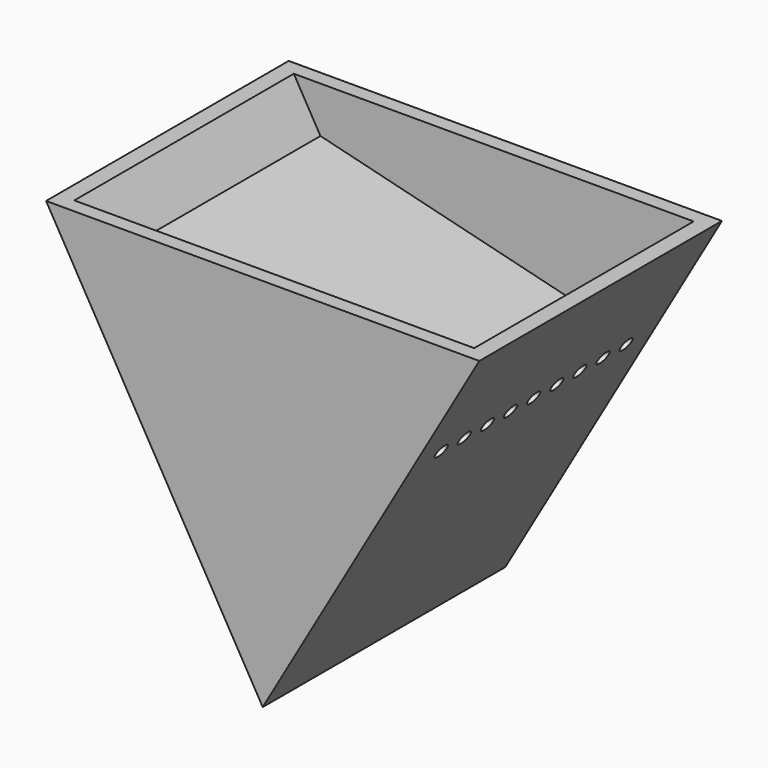
from build123d import *

# Parameters (mm, degrees)
F1_DEPTH = 105
F2_T     = -5
F4_DEPTH = 95
F6_D     = 5


with BuildPart() as f1:
    # F0 (on Front) → F1 (new body)
    with BuildSketch(Plane.XZ):
        Polygon((74.5727300216, 75.5225419998), (-75.4272699784, 75.5225419998), (-0.4272699784, -54.3812685678), align=None)
    extrude(amount=F1_DEPTH)

    # F2
    f2_openings = [f1.faces().sort_by_distance(p)[0] for p in [
        (-0.42727, -52.5, 75.522542),
    ]]
    offset(amount=F2_T, openings=f2_openings)

    # F3 (on face) → F4 (join)
    with BuildSketch(Plane.XZ.offset(5)):
        Polygon((44.5727300216, 33.5610177728), (-60.4272699784, 59.5417798863), (-0.4272699784, -44.3812685678), align=None)
    extrude(amount=F4_DEPTH)

    # F6 (through all)
    with Locations(Plane(origin=(18.8972005322, 0, -10.9103038142), x_dir=(0, -1, 0), z_dir=(-0.8660254038, 0, 0.5))):
        with Locations((92.5, 56.3510589789), (82.5, 56.3510589789), (72.5, 56.3510589789), (62.5, 56.3510589789), (52.5, 56.3510589789), (42.5, 56.3510589789), (32.5, 56.3510589789), (22.5, 56.3510589789), (12.5, 56.3510589789)):
            Hole(F6_D / 2)


solid = f1.part
